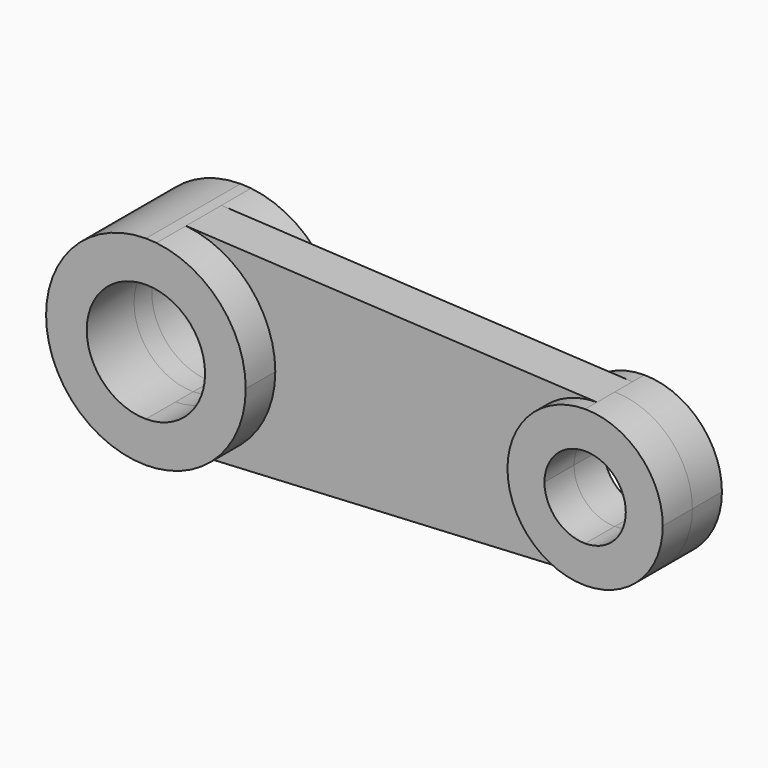
from build123d import *

# Parameters (mm, degrees)
F1_DEPTH = 25.4
F2_DEPTH = 25.4
F3_DEPTH = 9.525
F4_DEPTH = 9.525
F5_DEPTH = 15.875
F6_DEPTH = 15.875


with BuildPart() as f1:
    # F0 (on Front) → F1 (new body)
    with BuildSketch(Plane.XZ):
        with BuildLine():
            Line((0, 25.4), (0, 42.8625))
            ThreePointArc((0, 42.8625), (-42.8625, 0), (0, -42.8625))
            Line((0, -42.8625), (0, -25.4))
            ThreePointArc((0, -25.4), (-25.4, 0), (0, 25.4))
        make_face()
        with BuildLine():
            Line((4.499378453, 42.6256906077), (0, 42.8625))
            Line((0, 42.8625), (0, 25.4))
            ThreePointArc((0, 25.4), (17.9605122421, 17.9605122421), (25.4, 0))
            Line((25.4, 0), (42.8625, 0))
            ThreePointArc((42.8625, 0), (31.8594453435, 28.6735008092), (4.499378453, 42.6256906077))
        make_face()
        with BuildLine():
            Line((0, -25.4), (0, -42.8625))
            Line((0, -42.8625), (4.499378453, -42.6256906077))
            ThreePointArc((4.499378453, -42.6256906077), (31.8594453435, -28.6735008092), (42.8625, 0))
            Line((42.8625, 0), (25.4, 0))
            ThreePointArc((25.4, 0), (17.9605122421, -17.9605122421), (0, -25.4))
        make_face()
    extrude(amount=F1_DEPTH)

    # F2 (add): a face of the model
    f2_faces = [f1.faces().sort_by_distance(p)[0] for p in [
        (-41.6501654237, 0, 0),
    ]]
    extrude(f2_faces, amount=F2_DEPTH)

    # F0 (on Front) → F3 (join)
    with BuildSketch(Plane.XZ):
        with BuildLine():
            Line((0, -25.4), (0, -42.8625))
            Line((0, -42.8625), (4.499378453, -42.6256906077))
            ThreePointArc((4.499378453, -42.6256906077), (31.8594453435, -28.6735008092), (42.8625, 0))
            Line((42.8625, 0), (25.4, 0))
            ThreePointArc((25.4, 0), (17.9605122421, -17.9605122421), (0, -25.4))
        make_face()
        with BuildLine():
            Line((180.975, 33.3375), (4.499378453, 42.6256906077))
            ThreePointArc((4.499378453, 42.6256906077), (31.8594453435, 28.6735008092), (42.8625, 0))
            Line((42.8625, 0), (147.6375, 0))
            ThreePointArc((147.6375, 0), (157.4018276822, 23.5731723178), (180.975, 33.3375))
        make_face()
        with BuildLine():
            ThreePointArc((42.8625, 0), (31.8594453435, -28.6735008092), (4.499378453, -42.6256906077))
            Line((4.499378453, -42.6256906077), (180.975, -33.3375))
            ThreePointArc((180.975, -33.3375), (157.4018276822, -23.5731723178), (147.6375, 0))
            Line((147.6375, 0), (42.8625, 0))
        make_face()
    extrude(amount=F3_DEPTH)

    # F0 (on Front) → F4 (join)
    with BuildSketch(Plane.XZ):
        with BuildLine():
            Line((0, 25.4), (0, 42.8625))
            ThreePointArc((0, 42.8625), (-42.8625, 0), (0, -42.8625))
            Line((0, -42.8625), (0, -25.4))
            ThreePointArc((0, -25.4), (-25.4, 0), (0, 25.4))
        make_face()
        with BuildLine():
            Line((4.499378453, 42.6256906077), (0, 42.8625))
            Line((0, 42.8625), (0, 25.4))
            ThreePointArc((0, 25.4), (17.9605122421, 17.9605122421), (25.4, 0))
            Line((25.4, 0), (42.8625, 0))
            ThreePointArc((42.8625, 0), (31.8594453435, 28.6735008092), (4.499378453, 42.6256906077))
        make_face()
        with BuildLine():
            Line((0, -25.4), (0, -42.8625))
            Line((0, -42.8625), (4.499378453, -42.6256906077))
            ThreePointArc((4.499378453, -42.6256906077), (31.8594453435, -28.6735008092), (42.8625, 0))
            Line((42.8625, 0), (25.4, 0))
            ThreePointArc((25.4, 0), (17.9605122421, -17.9605122421), (0, -25.4))
        make_face()
        with BuildLine():
            Line((180.975, 33.3375), (4.499378453, 42.6256906077))
            ThreePointArc((4.499378453, 42.6256906077), (31.8594453435, 28.6735008092), (42.8625, 0))
            Line((42.8625, 0), (147.6375, 0))
            ThreePointArc((147.6375, 0), (157.4018276822, 23.5731723178), (180.975, 33.3375))
        make_face()
        with BuildLine():
            ThreePointArc((42.8625, 0), (31.8594453435, -28.6735008092), (4.499378453, -42.6256906077))
            Line((4.499378453, -42.6256906077), (180.975, -33.3375))
            ThreePointArc((180.975, -33.3375), (157.4018276822, -23.5731723178), (147.6375, 0))
            Line((147.6375, 0), (42.8625, 0))
        make_face()
    extrude(amount=-F4_DEPTH)

    # F0 (on Front) → F5 (join)
    with BuildSketch(Plane.XZ):
        with BuildLine():
            ThreePointArc((147.6375, 0), (157.4018276822, -23.5731723178), (180.975, -33.3375))
            Line((180.975, -33.3375), (180.975, -17.4625))
            ThreePointArc((180.975, -17.4625), (168.6271478335, -12.3478521665), (163.5125, 0))
            Line((163.5125, 0), (147.6375, 0))
        make_face()
        with BuildLine():
            Line((180.975, 17.4625), (180.975, 33.3375))
            ThreePointArc((180.975, 33.3375), (157.4018276822, 23.5731723178), (147.6375, 0))
            Line((147.6375, 0), (163.5125, 0))
            ThreePointArc((163.5125, 0), (168.6271478335, 12.3478521665), (180.975, 17.4625))
        make_face()
        with BuildLine():
            ThreePointArc((214.3125, 0), (204.5481723178, 23.5731723178), (180.975, 33.3375))
            Line((180.975, 33.3375), (180.975, 17.4625))
            ThreePointArc((180.975, 17.4625), (193.3228521665, 12.3478521665), (198.4375, 0))
            ThreePointArc((198.4375, 0), (193.3228521665, -12.3478521665), (180.975, -17.4625))
            Line((180.975, -17.4625), (180.975, -33.3375))
            ThreePointArc((180.975, -33.3375), (204.5481723178, -23.5731723178), (214.3125, 0))
        make_face()
    extrude(amount=F5_DEPTH)

    # F0 (on Front) → F6 (join)
    with BuildSketch(Plane.XZ):
        with BuildLine():
            ThreePointArc((147.6375, 0), (157.4018276822, -23.5731723178), (180.975, -33.3375))
            Line((180.975, -33.3375), (180.975, -17.4625))
            ThreePointArc((180.975, -17.4625), (168.6271478335, -12.3478521665), (163.5125, 0))
            Line((163.5125, 0), (147.6375, 0))
        make_face()
        with BuildLine():
            Line((180.975, 17.4625), (180.975, 33.3375))
            ThreePointArc((180.975, 33.3375), (157.4018276822, 23.5731723178), (147.6375, 0))
            Line((147.6375, 0), (163.5125, 0))
            ThreePointArc((163.5125, 0), (168.6271478335, 12.3478521665), (180.975, 17.4625))
        make_face()
        with BuildLine():
            ThreePointArc((214.3125, 0), (204.5481723178, 23.5731723178), (180.975, 33.3375))
            Line((180.975, 33.3375), (180.975, 17.4625))
            ThreePointArc((180.975, 17.4625), (193.3228521665, 12.3478521665), (198.4375, 0))
            ThreePointArc((198.4375, 0), (193.3228521665, -12.3478521665), (180.975, -17.4625))
            Line((180.975, -17.4625), (180.975, -33.3375))
            ThreePointArc((180.975, -33.3375), (204.5481723178, -23.5731723178), (214.3125, 0))
        make_face()
    extrude(amount=-F6_DEPTH)


solid = f1.part
